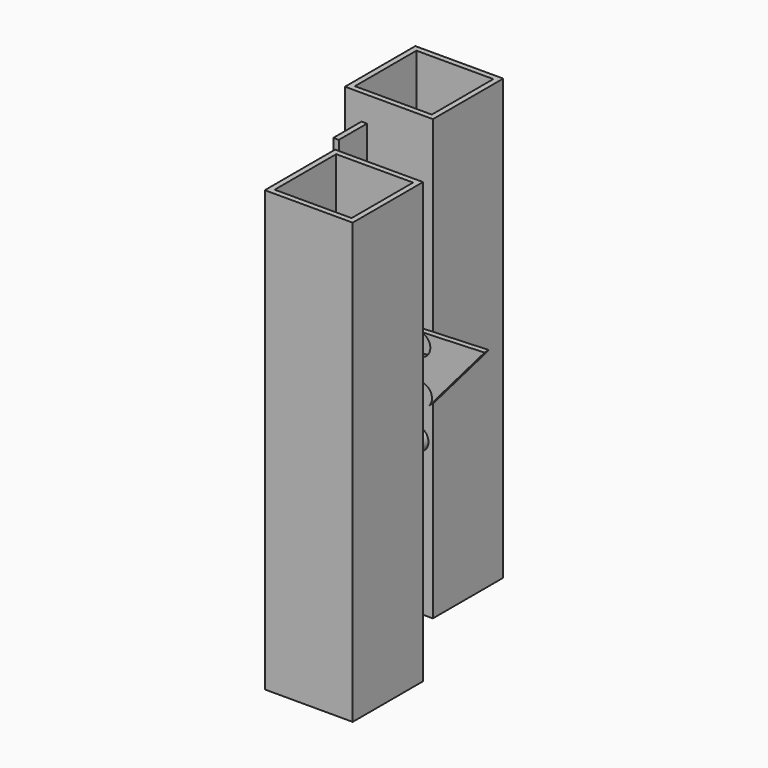
from build123d import *

# Parameters (mm, degrees)
F1_DEPTH  = 50.8
F2_R      = 3.175
F3_DEPTH  = 14.3202627102
F4_W      = 50.8
F4_H      = 50.8
F4_W_2    = 44.45
F4_H_2    = 44.45
F5_DEPTH  = 127
F6_R      = 6.35
F7_DEPTH  = 25.4
F8_R      = 6.35
F8_W      = 3.175
F8_H      = 25.4
F9_DEPTH  = 20.32
F11_START = 15.875
F10_R     = 3.81
F10_R_2   = 3.175
F11_DEPTH = 3.175
F12_START = 9.525
F8_W_2    = 31.75
F8_H_2    = 152.4
F8_R_2    = 7.62
F12_DEPTH = 9.525
F13_R     = 3.175
F13_R_2   = 1.5875
F14_DEPTH = 12.7
F15_R     = 6.35
F16_DEPTH = 31.75


# Not quite as in the source:
# - a feature names something its author has since deleted; it is built from what else it names


with BuildPart() as f1:
    # F0 (on Top) → F1 (new body)
    with BuildSketch(Plane.XY):
        with BuildLine():
            Line((0, 28.575), (0, 31.75))
            Line((0, 31.75), (-11.1442627102, 31.75))
            ThreePointArc((-11.1442627102, 31.75), (-9.940629285, 30.1852915304), (-8.7986979368, 28.575))
            Line((-8.7986979368, 28.575), (0, 28.575))
        make_face()
        Polygon((25.4, 28.575), (25.4, 31.75), (0, 31.75), (0, 28.575), (0, -28.575), (0, -31.75), (25.4, -31.75), (25.4, -28.575), (3.175, -28.575), (3.175, 28.575), align=None)
        with BuildLine():
            Line((0, -31.75), (0, -28.575))
            Line((0, -28.575), (-8.7986979368, -28.575))
            ThreePointArc((-8.7986979368, -28.575), (-9.940629285, -30.1852915304), (-11.1442627102, -31.75))
            Line((-11.1442627102, -31.75), (0, -31.75))
        make_face()
    extrude(amount=F1_DEPTH)

    # F2 (on face) → F3 (cut, through all)
    with BuildSketch(Plane.YZ.offset(3.175)):
        with Locations((0, 25.4)):
            Circle(F2_R)
    extrude(amount=-F3_DEPTH, mode=Mode.SUBTRACT)

    # F6 (on face) → F7 (join)
    with BuildSketch(Plane.XZ.offset(31.75)):
        with Locations((3.175, 25.4)):
            Circle(F6_R)
    extrude(amount=F7_DEPTH)


with BuildPart() as f5:
    # F4 (on Top) → F5 (new body, symmetric)
    with BuildSketch(Plane.XY):
        with Locations((28.575, 0)):
            Rectangle(F4_W, F4_H)
        with Locations((28.575, 0)):
            Rectangle(F4_W_2, F4_H_2, mode=Mode.SUBTRACT)
    extrude(amount=F5_DEPTH, both=True)

    # F8 (on face) → F9 (join)
    with BuildSketch(Plane.XZ.offset(25.4)):
        with Locations((34.925, 19.05)):
            Circle(F8_R)
        with Locations((14.2875, 99.6379471987)):
            Rectangle(F8_W, F8_H)
    extrude(amount=F9_DEPTH)


with BuildPart() as f5b:
    # F4 (on Top) → F5, piece 2 (new body, symmetric)
    with BuildSketch(Plane.XY):
        with Locations((63.5, -101.6)):
            Rectangle(F4_W, F4_H)
        with Locations((63.5, -101.6)):
            Rectangle(F4_W_2, F4_H_2, mode=Mode.SUBTRACT)
    extrude(amount=F5_DEPTH, both=True)

    # F15 (on face) → F16 (join)
    with BuildSketch(Plane(origin=(0, -76.2, 0), x_dir=(-1, 0, 0), z_dir=(0, 1, 0))):
        with Locations((-60.325, -25.4)):
            Circle(F15_R)
    extrude(amount=F16_DEPTH)


with BuildPart() as f11:
    # F10 (on face) → F11 (new body)
    with BuildSketch(Plane.XZ.offset(31.75).offset(F11_START)):
        with BuildLine():
            ThreePointArc((28.5750004077, 19.0532180694), (27.724261604, 15.8782178656), (25.4, 13.55395652))
            Line((25.4, 13.55395652), (25.4, 12.3489060883))
            Line((25.4, 12.3489060883), (68.0639762232, 8.0249561852))
            ThreePointArc((68.0639762232, 8.0249561852), (73.3180108307, 4.0694128265), (72.2496087167, -2.4197874203))
            Line((72.2496087167, -2.4197874203), (104.1447286146, 34.8758902287))
            Line((104.1447286146, 34.8758902287), (66.2178465005, 33.4344126184))
            ThreePointArc((66.2178465005, 33.4344126184), (72.8052703736, 26.8709436265), (65.7828861663, 20.7750926985))
            Line((65.7828861663, 20.7750926985), (25.4, 25.0995258416))
            Line((25.4, 25.0995258416), (25.4, 24.5524796189))
            ThreePointArc((25.4, 24.5524796189), (27.724261604, 22.2282182733), (28.5750004077, 19.0532180694))
        make_face()
        with Locations((44.4250904951, 16.6759039528)):
            Circle(F10_R, mode=Mode.SUBTRACT)
        with BuildLine():
            Line((25.4, 13.55395652), (25.4, 19.0532180694))
            Line((25.4, 19.0532180694), (25.4, 24.5524796189))
            ThreePointArc((25.4, 24.5524796189), (24.1931740543, 25.0905016057), (22.9011294955, 25.367119356))
            ThreePointArc((22.9011294955, 25.367119356), (15.9092059707, 19.7114282405), (21.5847144531, 12.7355813359))
            ThreePointArc((21.5847144531, 12.7355813359), (23.556776587, 12.8444442607), (25.4, 13.55395652))
        make_face()
        with Locations((22.2250004077, 19.0532180694)):
            Circle(F10_R_2, mode=Mode.SUBTRACT)
        with BuildLine():
            Line((25.4, 24.5524796189), (25.4, 19.0532180694))
            Line((25.4, 19.0532180694), (25.4, 13.55395652))
            ThreePointArc((25.4, 13.55395652), (27.724261604, 15.8782178656), (28.5750004077, 19.0532180694))
            ThreePointArc((28.5750004077, 19.0532180694), (27.724261604, 22.2282182733), (25.4, 24.5524796189))
        make_face()
        with BuildLine():
            Line((25.4, 13.55395652), (25.4, 19.0532180694))
            Line((25.4, 19.0532180694), (25.4, 24.5524796189))
            ThreePointArc((25.4, 24.5524796189), (24.1931740543, 25.0905016057), (22.9011294955, 25.367119356))
            ThreePointArc((22.9011294955, 25.367119356), (15.9092059707, 19.7114282405), (21.5847144531, 12.7355813359))
            ThreePointArc((21.5847144531, 12.7355813359), (23.556776587, 12.8444442607), (25.4, 13.55395652))
        make_face()
        with Locations((22.2250004077, 19.0532180694)):
            Circle(F10_R_2, mode=Mode.SUBTRACT)
        with BuildLine():
            ThreePointArc((22.9011294955, 25.367119356), (24.1931740543, 25.0905016057), (25.4, 24.5524796189))
            Line((25.4, 24.5524796189), (25.4, 25.0995258416))
            Line((25.4, 25.0995258416), (22.9011294955, 25.367119356))
        make_face()
        with BuildLine():
            Line((25.4, 12.3489060883), (25.4, 13.55395652))
            ThreePointArc((25.4, 13.55395652), (23.556776587, 12.8444442607), (21.5847144531, 12.7355813359))
            Line((21.5847144531, 12.7355813359), (25.4, 12.3489060883))
        make_face()
    extrude(amount=F11_DEPTH)


with BuildPart() as f12:
    # F8 (on face) → F12 (new body)
    with BuildSketch(Plane.XZ.offset(25.4).offset(F12_START)):
        with Locations((31.75, -38.1)):
            Rectangle(F8_W_2, F8_H_2)
        with Locations((34.925, 19.05)):
            Circle(F8_R_2, mode=Mode.SUBTRACT)
        with Locations((31.75, -38.1)):
            Rectangle(F8_W_2, F8_H_2)
        with Locations((34.925, 19.05)):
            Circle(F8_R_2, mode=Mode.SUBTRACT)
    extrude(amount=F12_DEPTH)

    # F13 (on face) → F14 (join)
    with BuildSketch(Plane.XZ.offset(44.45)):
        with Locations((22.225, 19.05)):
            Circle(F13_R)
        with Locations((44.6786, 15.24)):
            Circle(F13_R_2)
    extrude(amount=F14_DEPTH)


solid = Compound([f1.part, f5.part, f5b.part, f11.part, f12.part])
